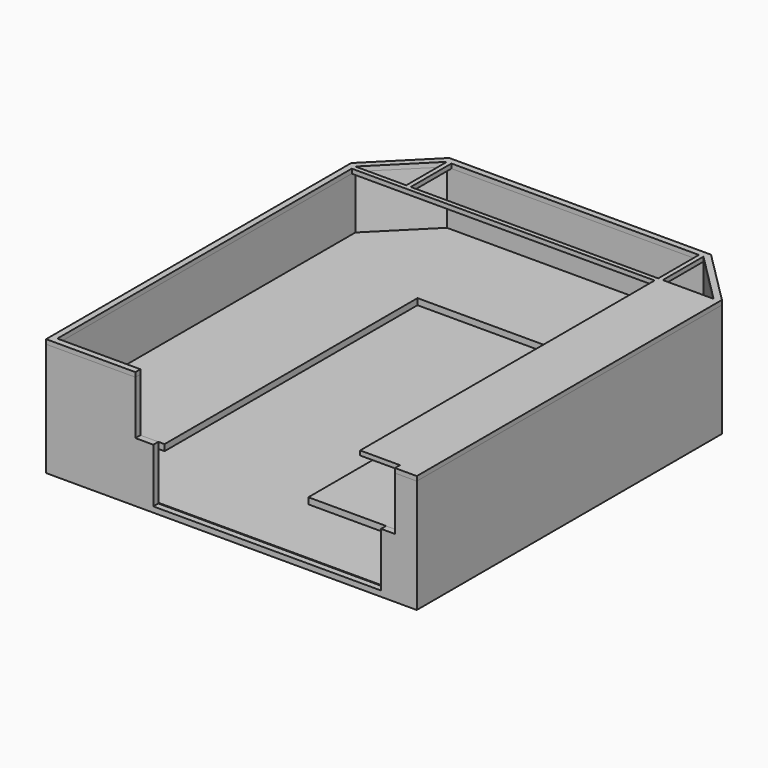
from build123d import *

# Parameters (mm, degrees)
F1_DEPTH  = 6350
F2_T      = -350
F3_W      = 12750
F3_H      = 3040
F4_DEPTH  = 350
F5_W      = 13852.0505063388
F5_H      = 254
F5_W_2    = 254
F5_H_2    = 20601.0252531694
F5_W_3    = 2844.9747468306
F5_H_3    = 2844.9747468306
F6_DEPTH  = 250
F7_W      = 3657.6
F7_H      = 4572
F8_DEPTH  = 914.4
F10_DEPTH = 300
F12_DEPTH = 350


# Not quite as in the source:
# - a feature names something its author has since deleted; it is built from what else it names


with BuildPart() as f1:
    # F0 (on Top) → F1 (new body)
    with BuildSketch(Plane.XY):
        Polygon((7325, 12200), (-7325, 12200), (-10375, 9150), (-10375, -12200), (10375, -12200), (10375, 9150), align=None)
    extrude(amount=F1_DEPTH)

    # F2
    f2_openings = [f1.faces().sort_by_distance(p)[0] for p in [
        (0, -209.322901, 6350),
    ]]
    offset(amount=F2_T, openings=f2_openings)

    # F3 (on face) → F4 (cut, through all)
    with BuildSketch(Plane.XZ.offset(12200)):
        with Locations((2000, 1830)):
            Rectangle(F3_W, F3_H)
        Polygon((9155, 6350), (-5375, 6350), (-5375, 3350), (-4375, 3350), (8375, 3350), (9155, 3350), align=None)
    extrude(amount=-F4_DEPTH, mode=Mode.SUBTRACT)

    # F7 (on face) → F8 (join)
    with BuildSketch(Plane(origin=(0, 0, 0), x_dir=(1, 0, 0), z_dir=(0, 0, -1))):
        with Locations((0, 6866)):
            Rectangle(F7_W, F7_H)
    extrude(amount=F8_DEPTH)


with BuildPart() as f6:
    # F5 (on face) → F6 (new body)
    with BuildSketch(Plane.XY.offset(6350)):
        Polygon((-7325, 12200), (-10375, 9150), (-10375, -12200), (-5375, -12200), (-5375, -11850), (-6926.0252531694, -11850), (-10025, -11850), (-10025, 8751.0252531694), (-10025, 9005.0252531694), (-7180.0252531694, 11850), (-6926.0252531694, 11850), (6926.0252531694, 11850), (7180.0252531694, 11850), (10025, 9005.0252531694), (10025, 8751.0252531694), (10025, -11850), (10375, -11850), (10375, 9150), (7325, 12200), align=None)
        Polygon((10375, -12200), (10375, -11850), (10025, -11850), (9155, -11850), (9155, -12200), align=None)
        with Locations((0, 8878.0252531694)):
            Rectangle(F5_W, F5_H)
        with Locations((-7053.0252531694, 8878.0252531694)):
            Rectangle(F5_W_2, F5_H)
        with Locations((7053.0252531694, -1549.4873734153)):
            Rectangle(F5_W_2, F5_H_2)
        Polygon((9155, -11850), (10025, -11850), (10025, 8751.0252531694), (7180.0252531694, 8751.0252531694), (7180.0252531694, -11850), align=None)
        with Locations((-8602.5126265847, 8878.0252531694)):
            Rectangle(F5_W_3, F5_H)
        with Locations((7053.0252531694, 8878.0252531694)):
            Rectangle(F5_W_2, F5_H)
        with Locations((-7053.0252531694, 10427.5126265847)):
            Rectangle(F5_W_2, F5_H_3)
        with Locations((8602.5126265847, 8878.0252531694)):
            Rectangle(F5_W_3, F5_H)
        with Locations((7053.0252531694, 10427.5126265847)):
            Rectangle(F5_W_2, F5_H_3)
    extrude(amount=F6_DEPTH)


with BuildPart() as f10:
    # F9 (on face) → F10 (new body)
    with BuildSketch(Plane.XY.offset(3350)):
        Polygon((-10025, 9005.0252531694), (-10025, -11850), (-5375, -11850), (-5148.2, -11850), (-5148.2, 6973.2), (5148.2, 6973.2), (5148.2, -11850), (10025, -11850), (10025, 9005.0252531694), (7180.0252531694, 11850), (-7180.0252531694, 11850), align=None)
    extrude(amount=-F10_DEPTH)


with BuildPart() as f12:
    # F11 (on face) → F12 (new body)
    with BuildSketch(Plane.XY.offset(3350)):
        Polygon((-10025, 9005.0252531694), (-10025, -11850), (-4025, -11850), (-4025, 5850), (4025, 5850), (4025, -11850), (10025, -11850), (10025, 9005.0252531694), (7180.0252531694, 11850), (-7180.0252531694, 11850), align=None)
    extrude(amount=-F12_DEPTH)


solid = Compound([f1.part, f6.part, f10.part, f12.part])
